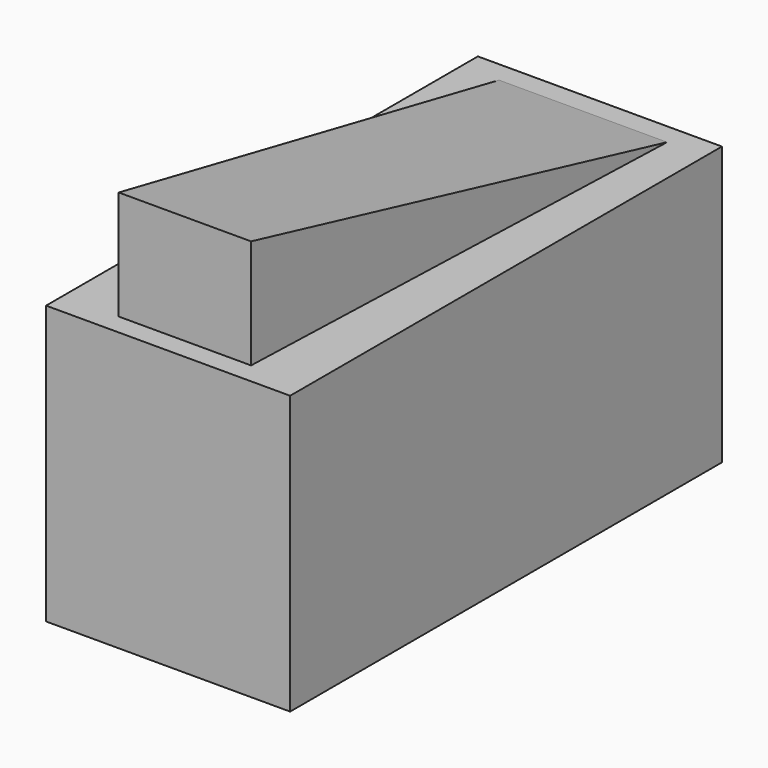
from build123d import *

# Parameters (mm, degrees)
F2_W     = 5.81
F2_H     = 12.85
F3_DEPTH = 6.62
F6_DEPTH = 2.6
F7_SIZE2 = 11.84999
F7_SIZE  = 2.59999


# Not quite as in the source:
# - a fillet or chamfer is up to 0.001 mm smaller than in the source, because OpenCascade refuses the exact size


with BuildPart() as f3:
    # F2 (on Top) → F3 (new body)
    with BuildSketch(Plane.XY):
        Rectangle(F2_W, F2_H)
    extrude(amount=F3_DEPTH)

    # F4 (on face) → F6 (join)
    with BuildSketch(Plane.XY.offset(6.62)):
        Polygon((2, 5.925), (-2, 5.925), (-1.575, -5.925), (1.575, -5.925), align=None)
    extrude(amount=F6_DEPTH)

    # F7 (size 2.6 and 11.85 in the source; OpenCascade refuses exactly that, so slightly less here)
    f7_edges = [f3.edges().sort_by_distance(p)[0] for p in [
        (0, 5.925, 9.22),
    ]]
    f7_side = f3.faces().sort_by_distance((0, 5.925, 7.92))[0]
    chamfer(f7_edges, length=F7_SIZE, length2=F7_SIZE2, reference=f7_side)


solid = f3.part
